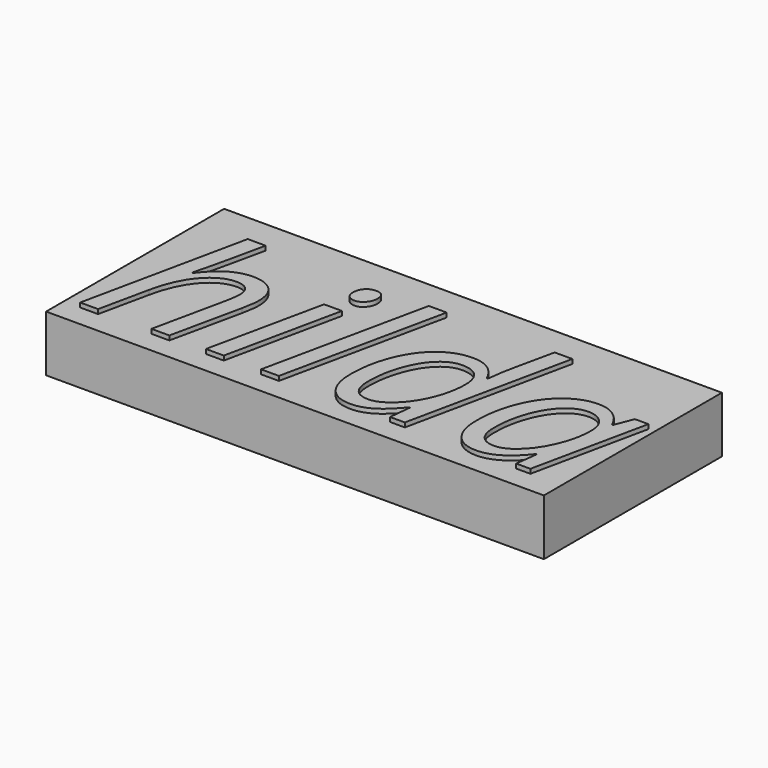
from build123d import *

# Parameters (mm, degrees)
F0_W         = 225.273668766
F0_H         = 100.7139757276
F1_DEPTH     = 25.4
F2_TEXT_SIZE = 98.5758987048
F3_DEPTH     = 2


# Not quite as in the source:
# - Text() gives the source's letters only with a copy of the font that has no kerning and outlines rounded to 1/6400 em; it was checked with that copy


with BuildPart() as f1:
    # F0 (on Top) → F1 (new body)
    with BuildSketch(Plane.XY):
        with Locations((112.636834383, 50.3569878638)):
            Rectangle(F0_W, F0_H)
    extrude(amount=F1_DEPTH)

    # F2 (on face) → F3 (join)
    with BuildSketch(Plane.XY.offset(25.4)):
        with Locations((4.6500009485, 9.9425101653)):
            Text('hilda', F2_TEXT_SIZE, font='Open Sans', font_style=FontStyle.ITALIC, text_align=(TextAlign.LEFT, TextAlign.BOTTOM))
    extrude(amount=F3_DEPTH)


solid = f1.part
